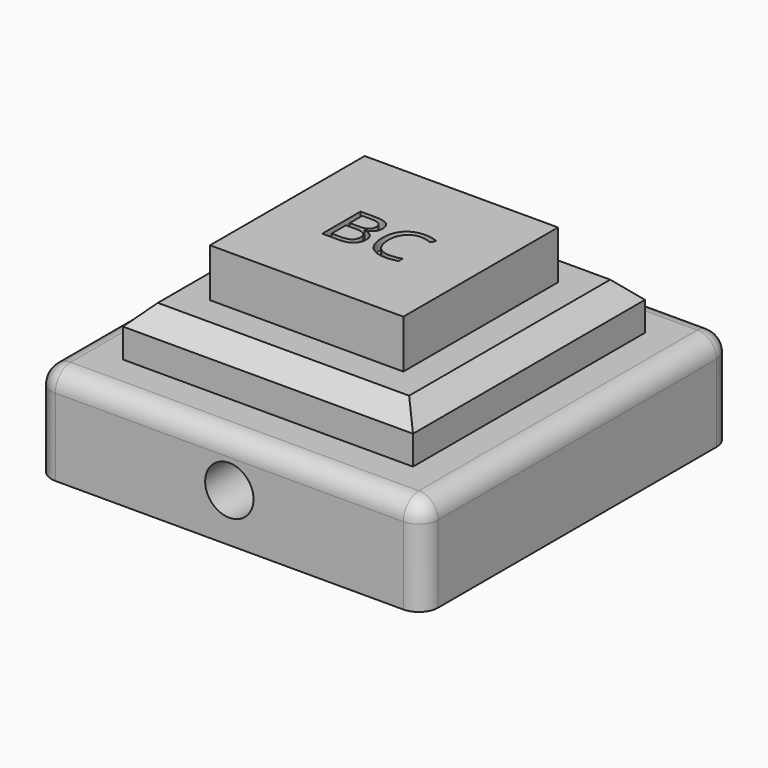
from build123d import *

# Parameters (mm, degrees)
F0_W          = 101.6
F0_H          = 101.6
F1_DEPTH      = 25.4
F2_W          = 76.2
F2_H          = 76.2
F3_DEPTH      = 12.7
F4_W          = 50.8
F4_H          = 50.8
F5_DEPTH      = 12.7
F6_R          = 6.35
F7_DEPTH      = 127
F8_R          = 5.08
F9_R          = 5.08
F10_R         = 5.08
F11_R         = 5.08
F12_SIZE      = 5.08
F13_SIZE      = 5.08
F14_SIZE      = 5.08
F15_SIZE      = 5.08
F16_TEXT_SIZE = 17.6388888889
F17_DEPTH     = 2.54


# Not quite as in the source:
# - Text() gives the source's letters only with a copy of the font that has no kerning and outlines rounded to 1/6400 em; it was checked with that copy


with BuildPart() as f1:
    # F0 (on Top) → F1 (new body)
    with BuildSketch(Plane.XY):
        with Locations((50.8, 50.8)):
            Rectangle(F0_W, F0_H)
    extrude(amount=F1_DEPTH)

    # F2 (on face) → F3 (join)
    with BuildSketch(Plane.XY.offset(25.4)):
        with Locations((50.8, 50.8)):
            Rectangle(F2_W, F2_H)
    extrude(amount=F3_DEPTH)

    # F4 (on face) → F5 (join)
    with BuildSketch(Plane.XY.offset(38.1)):
        with Locations((50.8, 50.8)):
            Rectangle(F4_W, F4_H)
    extrude(amount=F5_DEPTH)

    # F6 (on face) → F7 (cut)
    with BuildSketch(Plane.XZ):
        with Locations((50.8, 12.7)):
            Circle(F6_R)
    extrude(amount=-F7_DEPTH, mode=Mode.SUBTRACT)

    # F8
    f8_edges = [f1.edges().sort_by_distance(p)[0] for p in [
        (50.8, 0, 25.4),
    ]]
    fillet(f8_edges, radius=F8_R)

    # F9
    f9_edges = [f1.edges().sort_by_distance(p)[0] for p in [
        (0, 53.34, 25.4),
    ]]
    fillet(f9_edges, radius=F9_R)

    # F10
    f10_edges = [f1.edges().sort_by_distance(p)[0] for p in [
        (53.34, 101.6, 25.4),
    ]]
    fillet(f10_edges, radius=F10_R)

    # F11
    f11_edges = [f1.edges().sort_by_distance(p)[0] for p in [
        (101.6, 50.8, 25.4),
    ]]
    fillet(f11_edges, radius=F11_R)

    # F12
    f12_edges = [f1.edges().sort_by_distance(p)[0] for p in [
        (88.9, 50.8, 38.1),
    ]]
    chamfer(f12_edges, length=F12_SIZE)

    # F13
    f13_edges = [f1.edges().sort_by_distance(p)[0] for p in [
        (48.26, 88.9, 38.1),
    ]]
    chamfer(f13_edges, length=F13_SIZE)

    # F14
    f14_edges = [f1.edges().sort_by_distance(p)[0] for p in [
        (12.7, 48.26, 38.1),
    ]]
    chamfer(f14_edges, length=F14_SIZE)

    # F15
    f15_edges = [f1.edges().sort_by_distance(p)[0] for p in [
        (50.8, 12.7, 38.1),
    ]]
    chamfer(f15_edges, length=F15_SIZE)

    # F16 (on face) → F17 (cut)
    with BuildSketch(Plane.XY.offset(50.8)):
        with Locations((38.4292118107, 43.8170904836)):
            Text('BC', F16_TEXT_SIZE, font='Open Sans', text_align=(TextAlign.LEFT, TextAlign.BOTTOM))
    extrude(amount=-F17_DEPTH, mode=Mode.SUBTRACT)


solid = f1.part
